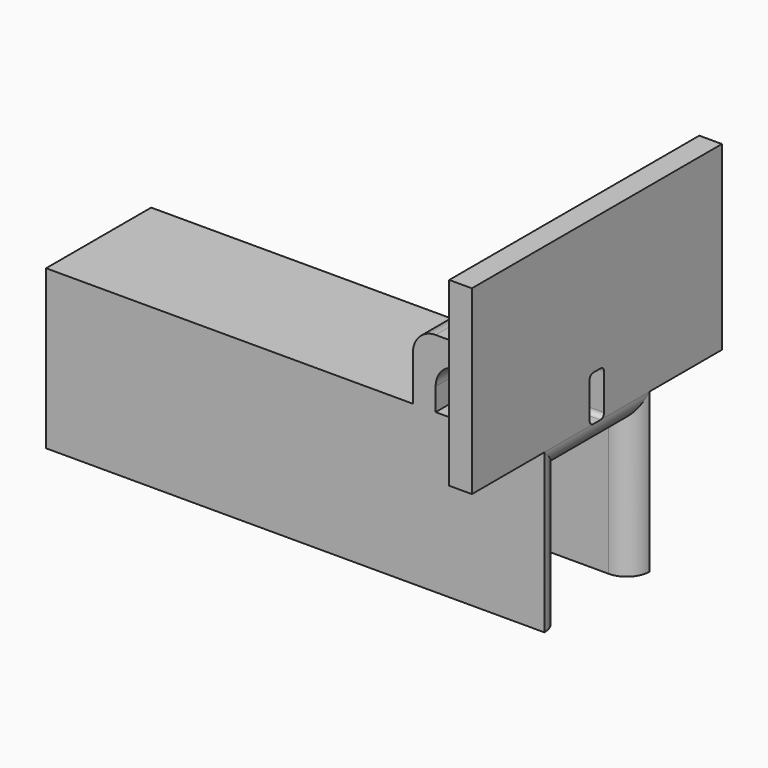
from build123d import *

# Parameters (mm, degrees)
F1_DEPTH = 110
F3_DEPTH = 5
F5_DEPTH = 29
F7_DEPTH = 5
F8_R     = 4.99999
F9_R     = 4.99999


# Not quite as in the source:
# - a fillet or chamfer is up to 0.001 mm smaller than in the source, because OpenCascade refuses the exact size


with BuildPart() as f1:
    # F0 (on Right) → F1 (new body)
    with BuildSketch(Plane.YZ):
        Polygon((-5, -30), (0, -30), (0, 0), (19, 0), (19, -30), (24, -30), (24, 5), (-5, 5), align=None)
    extrude(amount=-F1_DEPTH)

    # F2 (on face) → F3 (join)
    with BuildSketch(Plane.YZ):
        Polygon((-25, 5), (-5, 5), (24, 5), (44, 5), (44, 45), (-25, 45), align=None)
    extrude(amount=-F3_DEPTH)

    # F4 (on face) → F5 (join, through all)
    with BuildSketch(Plane.XZ.offset(5)):
        with BuildLine():
            Line((-19, 15), (-5, 15))
            Line((-5, 15), (-5, 20))
            Line((-5, 20), (-24, 20))
            ThreePointArc((-24, 20), (-27.5355339059, 18.5355339059), (-29, 15))
            Line((-29, 15), (-29, 5))
            Line((-29, 5), (-24, 5))
            Line((-24, 5), (-24, 10))
            ThreePointArc((-24, 10), (-22.5355339059, 13.5355339059), (-19, 15))
        make_face()
    extrude(amount=-F5_DEPTH)

    # F6 (on face) → F7 (cut, through all)
    with BuildSketch(Plane.YZ):
        with BuildLine():
            Line((8.5, 5), (9.5, 5))
            Line((9.5, 5), (10.5, 5))
            ThreePointArc((10.5, 5), (11.2071067812, 5.2928932188), (11.5, 6))
            Line((11.5, 6), (11.5, 14))
            ThreePointArc((11.5, 14), (11.2071067812, 14.7071067812), (10.5, 15))
            Line((10.5, 15), (8.5, 15))
            ThreePointArc((8.5, 15), (7.7928932188, 14.7071067812), (7.5, 14))
            Line((7.5, 14), (7.5, 6))
            ThreePointArc((7.5, 6), (7.7928932188, 5.2928932188), (8.5, 5))
        make_face()
    extrude(amount=-F7_DEPTH, mode=Mode.SUBTRACT)

    # F8 (radius 5 in the source; OpenCascade refuses exactly that, so slightly less here)
    f8_edges = [f1.edges().sort_by_distance(p)[0] for p in [
        (-110, 19, -15),
        (-110, 9.5, 0),
        (-110, 0, -15),
    ]]
    fillet(f8_edges, radius=F8_R)

    # F9 (radius 5 in the source; OpenCascade refuses exactly that, so slightly less here)
    f9_edges = [f1.edges().sort_by_distance(p)[0] for p in [
        (0, 0, -15),
        (0, 19, -15),
        (0, 9.5, 0),
    ]]
    fillet(f9_edges, radius=F9_R)


solid = f1.part
